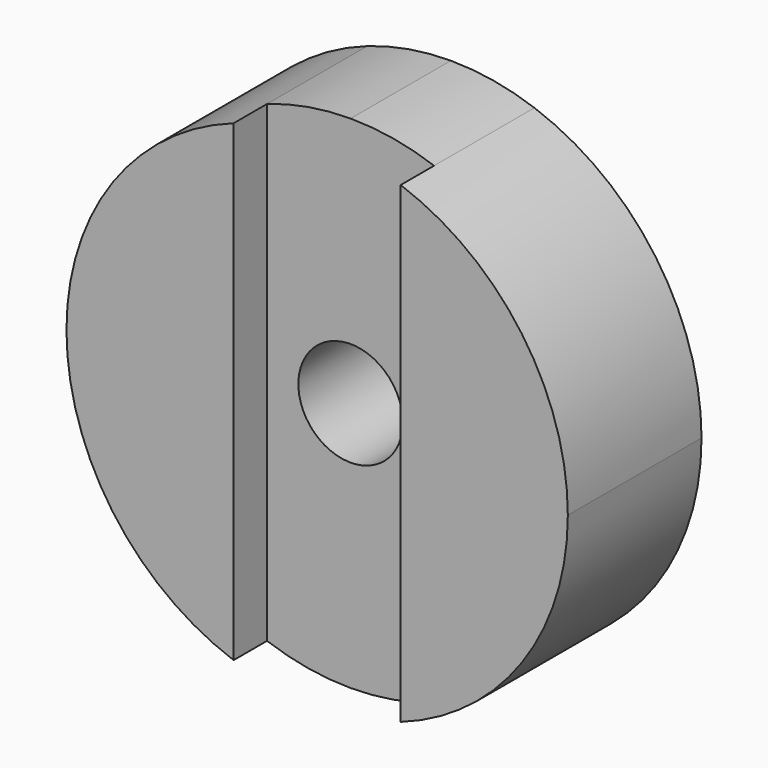
from build123d import *

# Parameters (mm, degrees)
F1_DEPTH = 12.7
F0_R     = 3.96875
F2_DEPTH = 9.525
F3_DEPTH = 62


# Not quite as in the source:
# - an extrude ends at something that could not be found from the text; its depth is read off the source's solid


with BuildPart() as f1:
    # F0 (on Front) → F1 (new body)
    with BuildSketch(Plane.XZ):
        with BuildLine():
            ThreePointArc((6.35, -17.9605122421), (15.5542598667, -10.9985226281), (19.05, 0))
            ThreePointArc((19.05, 0), (15.5542598667, 10.9985226281), (6.35, 17.9605122421))
            Line((6.35, 17.9605122421), (6.35, -17.9605122421))
        make_face()
    extrude(amount=F1_DEPTH)

    # F0 (on Front) → F3 (cut, through all)
    with BuildSketch(Plane.XZ):
        Circle(F0_R)
    extrude(amount=-F3_DEPTH, mode=Mode.SUBTRACT)


with BuildPart() as f1b:
    # F0 (on Front) → F1, piece 2 (new body)
    with BuildSketch(Plane.XZ):
        with BuildLine():
            Line((-6.35, -17.9605122421), (-6.35, 17.9605122421))
            ThreePointArc((-6.35, 17.9605122421), (-19.05, 0), (-6.35, -17.9605122421))
        make_face()
    extrude(amount=F1_DEPTH)


with BuildPart() as f2:
    # F0 (on Front) → F2 (new body)
    with BuildSketch(Plane.XZ):
        with BuildLine():
            Line((6.35, -17.9605122421), (6.35, 17.9605122421))
            ThreePointArc((6.35, 17.9605122421), (3.2213926947, 18.7756525614), (0, 19.05))
            ThreePointArc((0, 19.05), (-3.2213926947, 18.7756525614), (-6.35, 17.9605122421))
            Line((-6.35, 17.9605122421), (-6.35, -17.9605122421))
            ThreePointArc((-6.35, -17.9605122421), (-3.2213926947, -18.7756525614), (0, -19.05))
            ThreePointArc((0, -19.05), (3.2213926947, -18.7756525614), (6.35, -17.9605122421))
        make_face()
        Circle(F0_R, mode=Mode.SUBTRACT)
    extrude(amount=F2_DEPTH)


solid = Compound([f1.part, f1b.part, f2.part])
